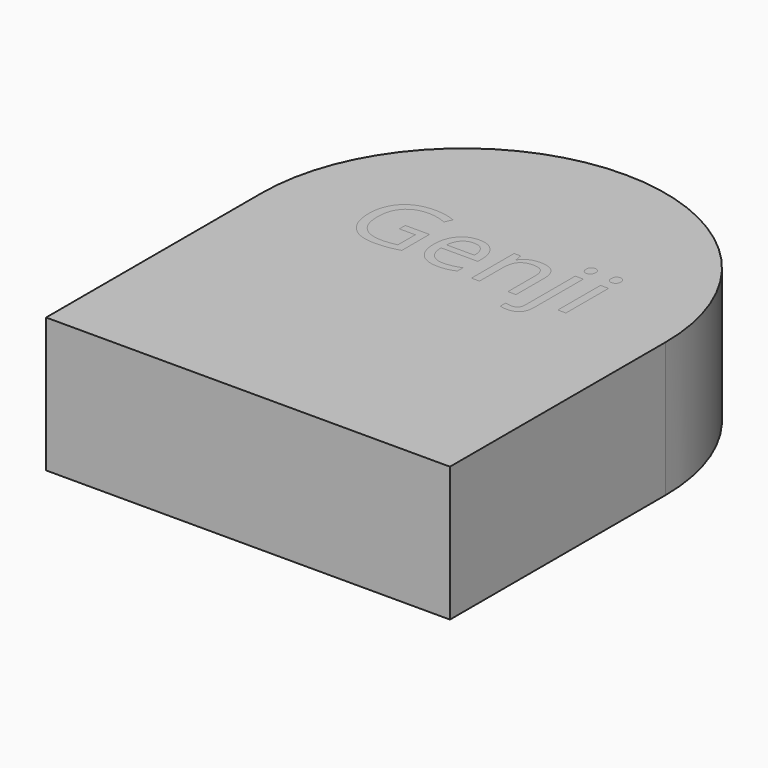
from build123d import *

# Parameters (mm, degrees)
F1_DEPTH     = 25.4
F2_TEXT_SIZE = 18.7993424738
F3_DEPTH     = 25.4


# Not quite as in the source:
# - Text() gives the source's letters only with a copy of the font that has no kerning and outlines rounded to 1/6400 em; it was checked with that copy


with BuildPart() as f1:
    # F0 (on Top) → F1 (new body)
    with BuildSketch(Plane.XY):
        with BuildLine():
            Line((-50.1315803215, 20.7932898068), (-50.1315803215, -30.0067101932))
            Line((-50.1315803215, -30.0067101932), (26.0684196785, -30.0067101932))
            Line((26.0684196785, -30.0067101932), (26.0684196785, 20.7932898068))
            ThreePointArc((26.0684196785, 20.7932898068), (-12.0315803215, 58.8932898068), (-50.1315803215, 20.7932898068))
        make_face()
    extrude(amount=F1_DEPTH)


with BuildPart() as f3:
    # F2 (on Top) → F3 (new body)
    with BuildSketch(Plane.XY):
        with Locations((-34.8915811628, 18.9497377723)):
            Text('Genji', F2_TEXT_SIZE, font='Open Sans', text_align=(TextAlign.LEFT, TextAlign.BOTTOM))
    extrude(amount=F3_DEPTH)


solid = Compound([f1.part, f3.part])
